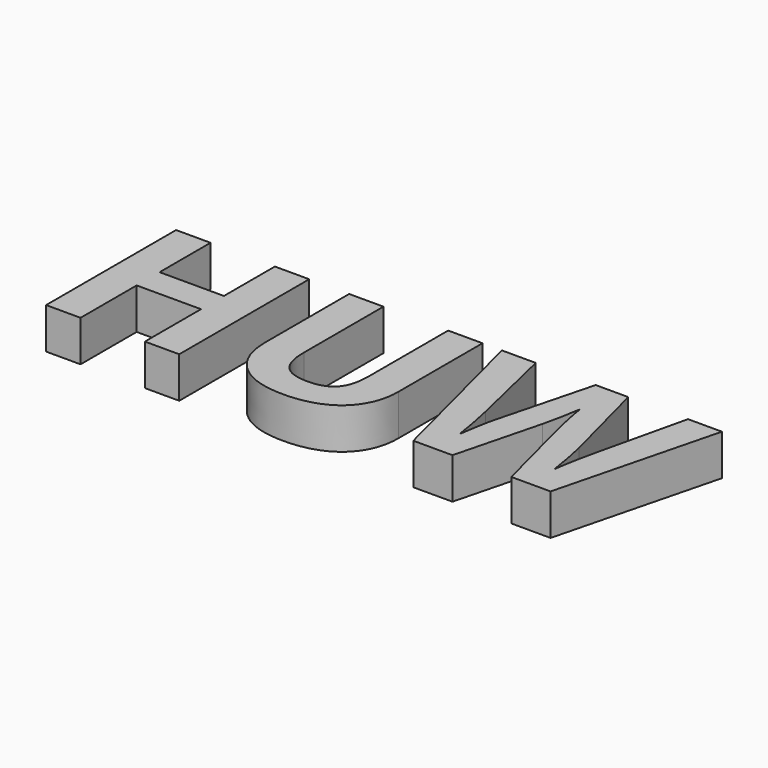
from build123d import *

# Parameters (mm, degrees)
F0_TEXT_SIZE = 11.1111111111
F1_DEPTH     = 2


# Not quite as in the source:
# - Text() gives the source's letters only with a copy of the font that has no kerning and outlines rounded to 1/6400 em; it was checked with that copy


with BuildPart() as f1:
    # F0 (on Top) → F1 (new body)
    with BuildSketch(Plane.XY):
        with Locations((-89.8718587815, -56.1958187544)):
            Text('HUW', F0_TEXT_SIZE, font='Open Sans', font_style=FontStyle.BOLD, text_align=(TextAlign.LEFT, TextAlign.BOTTOM))
    extrude(amount=F1_DEPTH)


solid = f1.part
